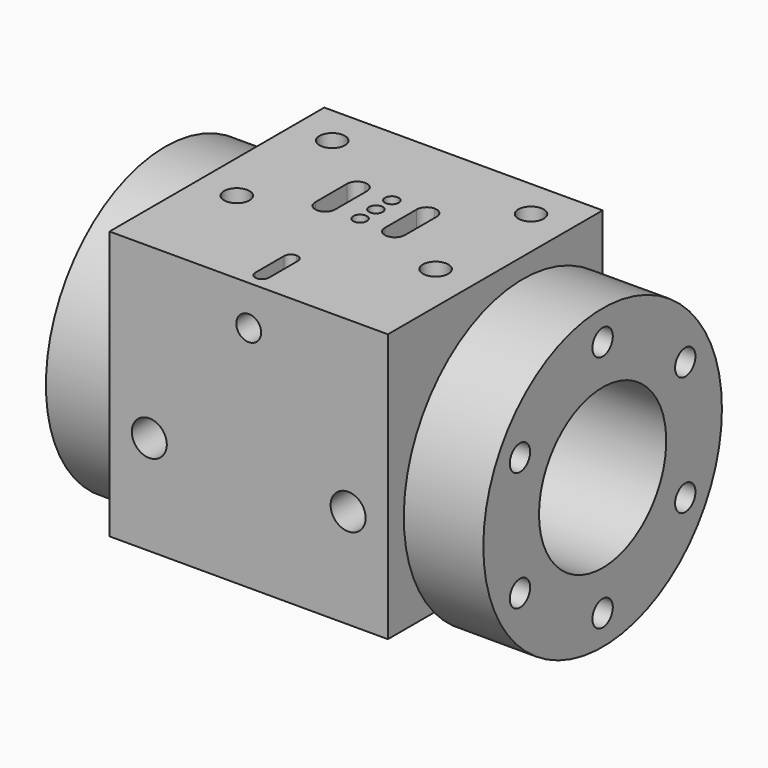
from build123d import *

# Parameters (mm, degrees)
F0_W             = 34.925
F0_H             = 25.4
F1_DEPTH         = 25.4
F3_DEPTH         = 6.35
F5_DEPTH         = 6.35
F6_D             = 12.7
F9_DEPTH         = 22.225
F11_D            = 2.794
F11_DEPTH        = 4.7625
F11_TIP          = 0.8394022848
F13_D            = 2.032
F13_DEPTH        = 4.7625
F13_TIP          = 0.6104743889
F16_D            = 2.032
F16_DEPTH        = 4.7625
F16_TIP          = 0.6104743889
F16_ON_F15_D     = 2.032
F16_ON_F15_DEPTH = 4.7625
F16_ON_F15_TIP   = 0.6104743889
F17_W            = 1.5875
F17_H            = 4.7625
F18_DEPTH        = 3.175
F19_R            = 0.79374
F20_R            = 0.9921875
F21_DEPTH        = 15.52488
F22_R            = 0.5461
F22_W            = 1.0922
F22_H            = 3.96875
F23_DEPTH        = 3.175
F24_R            = 0.54609


# Not quite as in the source:
# - a fillet or chamfer is up to 0.001 mm smaller than in the source, because OpenCascade refuses the exact size


with BuildPart() as f1:
    # F0 (on Top) → F1 (new body)
    with BuildSketch(Plane.XY):
        Rectangle(F0_W, F0_H)
    extrude(amount=F1_DEPTH)

    # F2 (on face) → F3 (cut)
    with BuildSketch(Plane.YZ.offset(17.4625)):
        with BuildLine():
            Line((-12.7, 25.4), (-12.7, 0))
            Line((-12.7, 0), (0.79375, 0))
            ThreePointArc((0.79375, 0), (-7.6252401135, 20.3252401135), (12.7, 11.90625))
            Line((12.7, 11.90625), (12.7, 25.4))
            Line((12.7, 25.4), (-12.7, 25.4))
        make_face()
        with BuildLine():
            ThreePointArc((12.7, 11.90625), (9.2127401135, 3.4872598865), (0.79375, 0))
            Line((0.79375, 0), (12.7, 0))
            Line((12.7, 0), (12.7, 11.90625))
        make_face()
    extrude(amount=-F3_DEPTH, mode=Mode.SUBTRACT)

    # F4 (on face) → F5 (cut)
    with BuildSketch(Plane(origin=(-17.4625, 0, 0), x_dir=(0, -1, 0), z_dir=(-1, 0, 0))):
        with BuildLine():
            ThreePointArc((11.1125, 11.90625), (7.6252401135, 3.4872598865), (-0.79375, 0))
            Line((-0.79375, 0), (12.7, 0))
            Line((12.7, 0), (12.7, 25.4))
            Line((12.7, 25.4), (-12.7, 25.4))
            Line((-12.7, 25.4), (-12.7, 11.9062500146))
            ThreePointArc((-12.7, 11.9062500146), (-0.7937499927, 23.8125), (11.1125, 11.90625))
        make_face()
        with BuildLine():
            Line((-12.7, 11.9062500146), (-12.7, 0))
            Line((-12.7, 0), (-0.79375, 0))
            ThreePointArc((-0.79375, 0), (-9.2127401186, 3.4872598916), (-12.7, 11.9062500146))
        make_face()
    extrude(amount=-F5_DEPTH, mode=Mode.SUBTRACT)

    # F6 (through all)
    with Locations(Plane.YZ.offset(17.4625)):
        with Locations((0.79375, 11.90625)):
            Hole(F6_D / 2)

    # F8 (on offset) → F9 (cut)
    with BuildSketch(Plane.YZ.offset(11.1125)):
        with BuildLine():
            Line((-12.7, 3.96875), (-12.7, 0))
            Line((-12.7, 0), (12.7, 0))
            Line((12.7, 0), (12.7, 25.4))
            Line((12.7, 25.4), (8.73125, 25.4))
            Line((8.73125, 25.4), (8.73125, 11.90625))
            ThreePointArc((8.73125, 11.90625), (6.4064100757, 6.2935899243), (0.79375, 3.96875))
            Line((0.79375, 3.96875), (-12.7, 3.96875))
        make_face()
    extrude(amount=-F9_DEPTH, mode=Mode.SUBTRACT)

    # F11
    with Locations(Plane.XZ.offset(12.7)):
        with Locations((-7.9375, 11.90625), (7.9375, 11.90625)):
            Hole(F11_D / 2, depth=F11_DEPTH)
            with Locations((0, 0, -(F11_DEPTH + F11_TIP / 2))):  # 118° drill point
                Cone(0, F11_D / 2, F11_TIP, mode=Mode.SUBTRACT)

    # F13
    with Locations(Plane.XY.offset(25.4)):
        with Locations((-7.9375, 5.55625), (7.9375, 5.55625), (7.9375, -3.96875), (-7.9375, -3.96875)):
            Hole(F13_D / 2, depth=F13_DEPTH)
            with Locations((0, 0, -(F13_DEPTH + F13_TIP / 2))):  # 118° drill point
                Cone(0, F13_D / 2, F13_TIP, mode=Mode.SUBTRACT)

    # F16
    with Locations(Plane.YZ.offset(17.4625)):
        with Locations((0.79375, 21.43125), (9.0426419749, 16.6687499934), (9.0426419634, 7.1437499867), (0.793749977, 2.38125), (-7.4551419864, 7.1437500265), (-7.4551419519, 16.6687500331)):
            Hole(F16_D / 2, depth=F16_DEPTH)
            with Locations((0, 0, -(F16_DEPTH + F16_TIP / 2))):  # 118° drill point
                Cone(0, F16_D / 2, F16_TIP, mode=Mode.SUBTRACT)

    # F16 on F15
    with Locations(Plane(origin=(-17.4625, 0, 0), x_dir=(0, -1, 0), z_dir=(-1, 0, 0))):
        with Locations((-0.79375, 21.43125), (-9.042641971, 16.66875), (-9.042641971, 7.14375), (-0.79375, 2.38125), (7.455141971, 7.14375), (7.455141971, 16.66875)):
            Hole(F16_ON_F15_D / 2, depth=F16_ON_F15_DEPTH)
            with Locations((0, 0, -(F16_ON_F15_DEPTH + F16_ON_F15_TIP / 2))):  # 118° drill point
                Cone(0, F16_ON_F15_D / 2, F16_ON_F15_TIP, mode=Mode.SUBTRACT)

    # F17 (on face) → F18 (cut)
    with BuildSketch(Plane.XY.offset(25.4)):
        with Locations((2.778125, 0)):
            Rectangle(F17_W, F17_H)
        with Locations((-2.778125, 0)):
            Rectangle(F17_W, F17_H)
    extrude(amount=-F18_DEPTH, mode=Mode.SUBTRACT)

    # F19 (radius 0.79375 in the source; OpenCascade refuses exactly that, so slightly less here)
    f19_edges = [f1.edges().sort_by_distance(p)[0] for p in [
        (-3.571875, 2.38125, 23.8125),
        (-1.984375, 2.38125, 23.8125),
        (-1.984375, -2.38125, 23.8125),
        (-3.571875, -2.38125, 23.8125),
        (1.984375, -2.38125, 23.8125),
        (3.571875, 2.38125, 23.8125),
        (1.984375, 2.38125, 23.8125),
        (3.571875, -2.38125, 23.8125),
    ]]
    fillet(f19_edges, radius=F19_R)

    # F20 (on face) → F21 (cut)
    with BuildSketch(Plane.XZ.offset(12.7)):
        with Locations((0, 22.225)):
            Circle(F20_R)
    extrude(amount=-F21_DEPTH, mode=Mode.SUBTRACT)

    # F22 (on face) → F23 (cut)
    with BuildSketch(Plane.XY.offset(25.4)):
        Circle(F22_R)
        with Locations((0, 1.5875)):
            Circle(F22_R)
        with Locations((0, -1.5875)):
            Circle(F22_R)
        with Locations((0, -9.921875)):
            Rectangle(F22_W, F22_H)
    extrude(amount=-F23_DEPTH, mode=Mode.SUBTRACT)

    # F24 (radius 0.5461 in the source; OpenCascade refuses exactly that, so slightly less here)
    f24_edges = [f1.edges().sort_by_distance(p)[0] for p in [
        (-0.5461, -7.9375, 24.226689),
        (0.5461, -7.9375, 24.226689),
        (0.5461, -11.90625, 24.226689),
        (-0.5461, -11.90625, 24.226689),
    ]]
    fillet(f24_edges, radius=F24_R)


solid = f1.part
